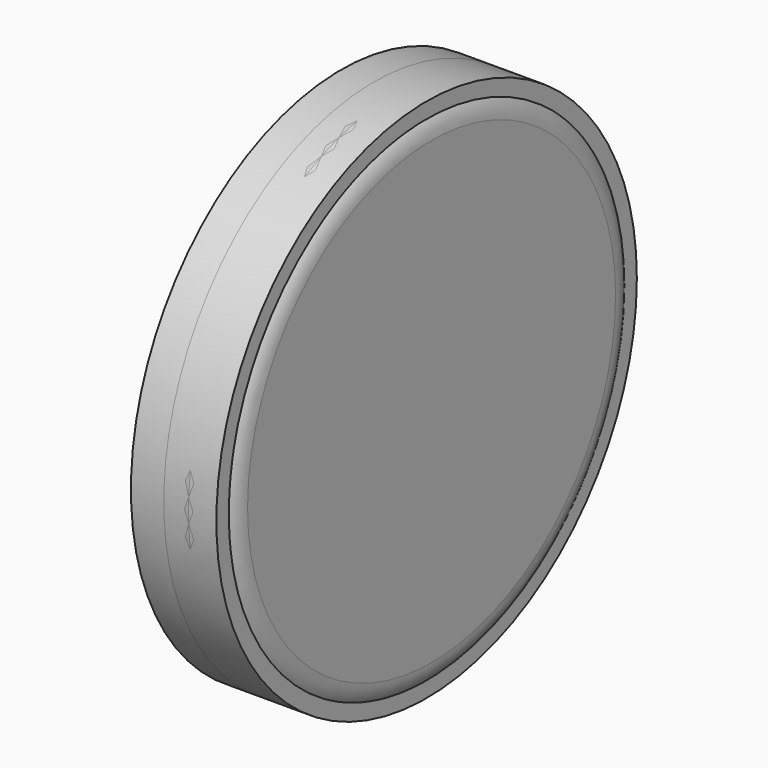
from build123d import *

# Parameters (mm, degrees)
F0_R      = 11
F1_DEPTH  = 1
F2_R      = 1
F3_DEPTH  = 2
F4_R      = 1
F5_R      = 16
F6_DEPTH  = 3.5
F7_DEPTH  = 0.5
F8_R      = 1.99999
F9_DEPTH  = 2
F10_DEPTH = 25
F12_R     = 16
F12_R_2   = 10.75
F13_DEPTH = 3.2


# Not quite as in the source:
# - a fillet or chamfer is up to 0.001 mm smaller than in the source, because OpenCascade refuses the exact size


with BuildPart() as f1:
    # F0 (on Right) → F1 (new body)
    with BuildSketch(Plane.YZ):
        Circle(F0_R)
    extrude(amount=F1_DEPTH)

    # F2 (on face) → F3 (join)
    with BuildSketch(Plane.YZ.offset(1)):
        with Locations((-6.2765460461, 7.0736445487)):
            Circle(F2_R)
    extrude(amount=F3_DEPTH)

    # F4
    f4_edges = [f1.edges().sort_by_distance(p)[0] for p in [
        (3, -7.276546, 7.073645),
    ]]
    fillet(f4_edges, radius=F4_R)


with BuildPart() as f6:
    # F5 (on Right) → F6 (new body)
    with BuildSketch(Plane.YZ):
        Circle(F5_R)
    extrude(amount=F6_DEPTH)

    # F7 (add): a face of the model
    f7_faces = [f6.faces().sort_by_distance(p)[0] for p in [
        (0, 0, 0),
    ]]
    extrude(f7_faces, amount=F7_DEPTH)

    # F8 (radius 2 in the source; OpenCascade refuses exactly that, so slightly less here)
    f8_edges = [f6.edges().sort_by_distance(p)[0] for p in [
        (3.5, -16, 0),
        (-0.5, -16, 0),
    ]]
    fillet(f8_edges, radius=F8_R)


with BuildPart() as f9:
    # F5 (on Right) → F9 (new body)
    with BuildSketch(Plane.YZ):
        Circle(F5_R)
    extrude(amount=-F9_DEPTH)


with BuildPart() as f10:
    # F5 (on Right) → F10 (new body)
    with BuildSketch(Plane.YZ):
        Circle(F5_R)
    extrude(amount=F10_DEPTH)


with BuildPart() as f13:
    # F12 (on face) → F13 (new body)
    with BuildSketch(Plane.YZ):
        Circle(F12_R)
        Circle(F12_R_2, mode=Mode.SUBTRACT)
    extrude(amount=F13_DEPTH)


solid = Compound([f1.part, f6.part, f9.part, f13.part])
